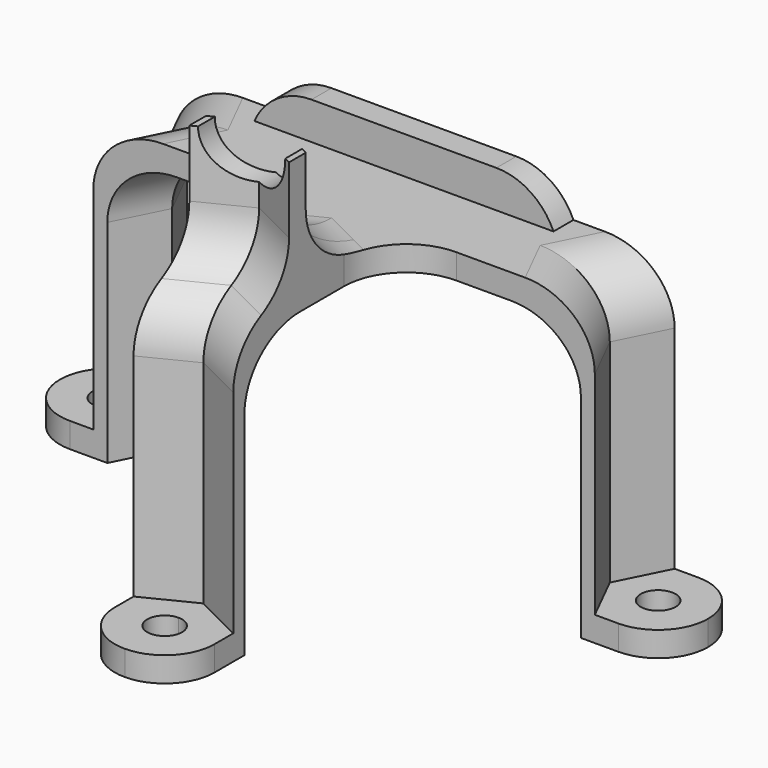
from build123d import *

# Parameters (mm, degrees)
F0_R         = 1.4
F1_DEPTH     = 2
F3_DEPTH     = 20
F5_DEPTH     = 2
F6_W         = 24.2574699223
F6_H         = 65.0979466736
F7_DEPTH     = 25
F8_R         = 5
F10_DEPTH    = 9
F11_R        = 5
F12_W        = 12
F12_H        = 2
F13_DEPTH    = 3
F14_T1_DEPTH = 24.9128784748
F16_R        = 3.5
F17_DEPTH    = 25


# Not quite as in the source:
# - a fillet or chamfer that OpenCascade refuses, or shapes differently, is made with other operations: its cross-section is extruded or revolved along the edge and cut away or added


with BuildPart() as f1:
    # F0 (on Top) → F1 (new body)
    with BuildSketch(Plane.XY):
        with BuildLine():
            ThreePointArc((22, -4), (24.8284271247, -2.8284271247), (26, 0))
            ThreePointArc((26, 0), (24.8284271247, 2.8284271247), (22, 4))
            ThreePointArc((22, 4), (18, 0), (22, -4))
        make_face()
        with Locations((22, 0)):
            Circle(F0_R, mode=Mode.SUBTRACT)
        with BuildLine():
            ThreePointArc((22, -4), (18, 0), (22, 4))
            Line((22, 4), (19, 4))
            Line((19, 4), (17, 0))
            Line((17, 0), (19, -4))
            Line((19, -4), (22, -4))
        make_face()
    extrude(amount=F1_DEPTH)

    # F2 (on face) → F3 (join)
    with BuildSketch(Plane.XY.offset(2)):
        Polygon((19, 4), (17, 0), (19, -4), (20.1180339887, -4), (18.1180339887, 0), (20.1180339887, 4), align=None)
    extrude(amount=F3_DEPTH)



with BuildPart() as f1b:
    # F0 (on Top) → F1, piece 2 (new body)
    with BuildSketch(Plane.XY):
        with BuildLine():
            ThreePointArc((-4, -22), (0, -26), (4, -22))
            ThreePointArc((4, -22), (0, -18), (-4, -22))
        make_face()
        with Locations((0, -22)):
            Circle(F0_R, mode=Mode.SUBTRACT)
        with BuildLine():
            ThreePointArc((-4, -22), (0, -18), (4, -22))
            Line((4, -22), (4, -19))
            Line((4, -19), (0, -17))
            Line((0, -17), (-4, -19))
            Line((-4, -19), (-4, -22))
        make_face()
    extrude(amount=F1_DEPTH)

    # F2 (on face) → F3, piece 2 (join)
    with BuildSketch(Plane.XY.offset(2)):
        Polygon((4, -19), (0, -17), (-4, -19), (-4, -20.1180339887), (0, -18.1180339887), (4, -20.1180339887), align=None)
    extrude(amount=F3_DEPTH)


with BuildPart() as f1_1:
    add(f1.part)

    add(f1b.part)  # F5 merges F1b
    # F4 (on face) → F5 (join)
    with BuildSketch(Plane.XY.offset(22)):
        Polygon((4, -20.1180339887), (4, -4), (0, -4), (0, -18.1180339887), align=None)
        Polygon((17, 0), (19, 4), (0, 4), (0, -4), (4, -4), (19, -4), align=None)
        Polygon((18.1180339887, 0), (20.1180339887, 4), (19, 4), (17, 0), (19, -4), (20.1180339887, -4), align=None)
    extrude(amount=F5_DEPTH)

    # F6 (on face) → F7 (cut)
    with BuildSketch(Plane.XY.offset(24)):
        with Locations((-12.1287349612, -10.913932696)):
            Rectangle(F6_W, F6_H)
    extrude(amount=-F7_DEPTH, mode=Mode.SUBTRACT)

    # F8
    f8_edges = [f1_1.edges().sort_by_distance(p)[0] for p in [
        (4, -4, 23),
        (2, -18, 22),
        (18, -2, 22),
        (18, 2, 22),
        (19.118034, -2, 24),
        (19.118034, 2, 24),
        (2, -19.118034, 24),
    ]]
    fillet(f8_edges, radius=F8_R)

    # F9 (on face) → F10 (join)
    with BuildSketch(Plane.XY.offset(24)):
        Polygon((0, -10.8508134726), (0, -12.527864045), (4, -14.527864045), (4, -12.8508134726), (0.6708202289, -11.1862235871), align=None)
    extrude(amount=F10_DEPTH)

    # F11
    f11_edges = [f1_1.edges().sort_by_distance(p)[0] for p in [
        (2, -11.850813, 24),
        (2, -13.527864, 24),
    ]]
    fillet(f11_edges, radius=F11_R)

    # F12 (on face) → F13 (join)
    with BuildSketch(Plane.XY.offset(24)):
        with Locations((6, 3)):
            Rectangle(F12_W, F12_H)
    extrude(amount=F13_DEPTH)

    # F14: fillet of radius 5 on 1 edges, made by hand

    # F14_s2 → F14_t1 (cut)
    with BuildSketch(Plane.XZ.offset(-15.4564392374)):
        with BuildLine():
            ThreePointArc((12, 24), (10.1560370926, 26.1833001327), (7.417424305, 27))
            Line((7.417424305, 27), (12, 27))
            Line((12, 27), (12, 24))
        make_face()
    extrude(amount=F14_T1_DEPTH, mode=Mode.SUBTRACT)

    # F15: F1 across face


with BuildPart() as f1_2:
    add(f1_1.part)
    add(f1_1.part.mirror(Plane(origin=(0, -10.4635359507, 20.0753373273), x_dir=(0, -1, 0), z_dir=(-1, 0, 0))))

    # F16 (on face) → F17 (cut)
    with BuildSketch(Plane(origin=(0, 4, 0), x_dir=(-1, 0, 0), z_dir=(0, 1, 0))):
        with Locations((0, 33)):
            Circle(F16_R)
    extrude(amount=-F17_DEPTH, mode=Mode.SUBTRACT)


solid = f1_2.part
